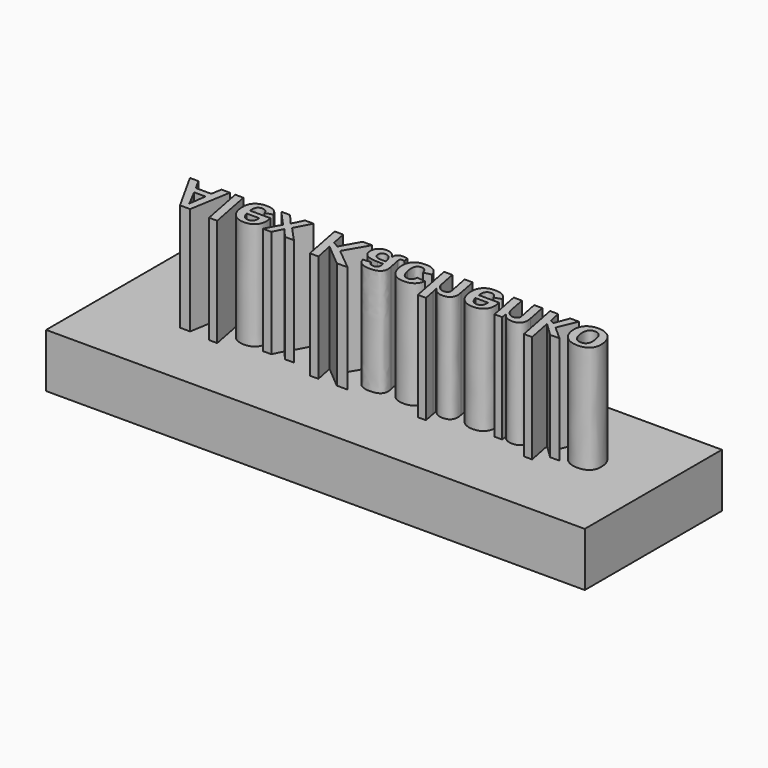
from build123d import *

# Parameters (mm, degrees)
F0_W         = 63.5
F0_H         = 20.2066265047
F1_DEPTH     = 6.35
F2_TEXT_SIZE = 7.0296216216
F3_DEPTH     = 19.05


# Not quite as in the source:
# - Text() gives the source's letters only with a copy of the font that has no kerning and outlines rounded to 1/6400 em; it was checked with that copy


with BuildPart() as f1:
    # F0 (on Top) → F1 (new body)
    with BuildSketch(Plane.XY):
        Rectangle(F0_W, F0_H)
    extrude(amount=F1_DEPTH)

    # F2 (on face) → F3 (join)
    with BuildSketch(Plane(origin=(0, 0, 0), x_dir=(1, 0, 0), z_dir=(0, 0, -1))):
        with Locations((-24.9502519662, -2.7698839697)):
            Text('Alex Kachenko', F2_TEXT_SIZE, font='Arimo', font_style=FontStyle.BOLDITALIC, text_align=(TextAlign.LEFT, TextAlign.BOTTOM))
    extrude(amount=-F3_DEPTH)


solid = f1.part
